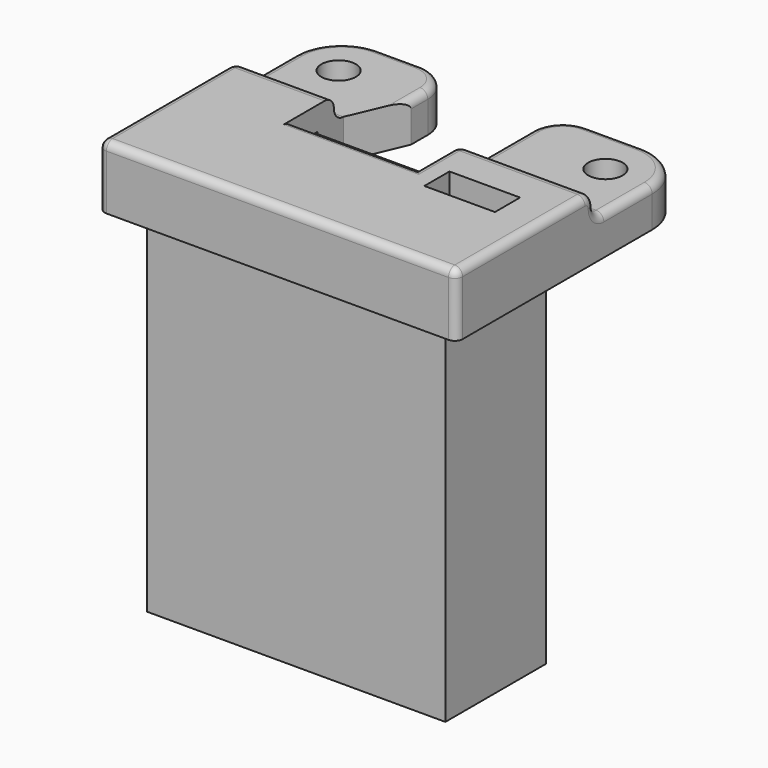
from build123d import *

# Parameters (mm, degrees)
F0_W      = 19
F0_H      = 8
F1_DEPTH  = 25
F2_W      = 22.8
F2_H      = 11
F3_DEPTH  = 1.5
F5_DEPTH  = 2.5
F6_R      = 1.1
F7_DEPTH  = 2.5
F8_R      = 0.74999
F10_DEPTH = 12.5
F11_R     = 2
F12_W     = 4.5
F12_H     = 2
F13_DEPTH = 25
F14_R     = 0.5
F15_R     = 0.5
F16_R     = 0.5


# Not quite as in the source:
# - a fillet or chamfer is up to 0.001 mm smaller than in the source, because OpenCascade refuses the exact size


with BuildPart() as f1:
    # F0 (on Top) → F1 (new body)
    with BuildSketch(Plane.XY):
        with Locations((0, 4)):
            Rectangle(F0_W, F0_H)
    extrude(amount=-F1_DEPTH)


with BuildPart() as f3:
    # F2 (on Top) → F3 (new body)
    with BuildSketch(Plane.XY):
        with Locations((0, 4)):
            Rectangle(F2_W, F2_H)
    extrude(amount=F3_DEPTH)

    # F4 (on face) → F5 (join)
    with BuildSketch(Plane(origin=(0, 0, 0), x_dir=(1, 0, 0), z_dir=(0, 0, -1))):
        Polygon((9.7, -9.5), (11.4, -9.5), (11.4, 1.5), (-11.4, 1.5), (-11.4, -9.5), (-9.7, -9.5), (-9.7, 0.2), (9.7, 0.2), align=None)
    extrude(amount=F5_DEPTH)

    # F6 (on face) → F7 (join)
    with BuildSketch(Plane(origin=(0, 0, 0), x_dir=(1, 0, 0), z_dir=(0, 0, -1))):
        with BuildLine():
            Line((11.4, -14.1), (11.4, -8.2))
            Line((11.4, -8.2), (-11.4, -8.2))
            Line((-11.4, -8.2), (-11.4, -14.1))
            ThreePointArc((-11.4, -14.1), (-10.5213203436, -16.2213203436), (-8.4, -17.1))
            Line((-8.4, -17.1), (8.4, -17.1))
            ThreePointArc((8.4, -17.1), (10.5213203436, -16.2213203436), (11.4, -14.1))
        make_face()
        with Locations((-8.5, -14)):
            Circle(F6_R, mode=Mode.SUBTRACT)
        with Locations((8.5, -14)):
            Circle(F6_R, mode=Mode.SUBTRACT)
    extrude(amount=F7_DEPTH)

    # F8 (radius 0.75 in the source; OpenCascade refuses exactly that, so slightly less here)
    f8_edges = [f3.edges().sort_by_distance(p)[0] for p in [
        (0, 9.5, 0),
        (0, 9.5, 1.5),
    ]]
    fillet(f8_edges, radius=F8_R)

    # F9 (on Top) → F10 (cut, symmetric)
    with BuildSketch(Plane.XY):
        Polygon((2.9, 6), (2.9, 23.4100954436), (-3.7, 23.4100954436), (-3.7, 13.75), (-5.2, 10.25), (-5.2, 6), align=None)
    extrude(amount=F10_DEPTH, both=True, mode=Mode.SUBTRACT)

    # F11
    f11_edges = [f3.edges().sort_by_distance(p)[0] for p in [
        (-3.7, 17.1, -1.25),
        (2.9, 17.1, -1.25),
    ]]
    fillet(f11_edges, radius=F11_R)

    # F12 (on face) → F13 (cut)
    with BuildSketch(Plane.XY.offset(1.5)):
        with Locations((6.65, 5.7)):
            Rectangle(F12_W, F12_H)
    extrude(amount=-F13_DEPTH, mode=Mode.SUBTRACT)

    # F14
    f14_edges = [f3.edges().sort_by_distance(p)[0] for p in [
        (11.4, -1.5, -0.5),
        (-11.4, -1.5, -0.5),
    ]]
    fillet(f14_edges, radius=F14_R)

    # F15
    f15_edges = [f3.edges().sort_by_distance(p)[0] for p in [
        (11.4, 3.875005, 1.5),
    ]]
    fillet(f15_edges, radius=F15_R)

    # F16
    f16_edges = [f3.edges().sort_by_distance(p)[0] for p in [
        (-1.15, 6, 1.5),
    ]]
    fillet(f16_edges, radius=F16_R)


solid = Compound([f1.part, f3.part])
